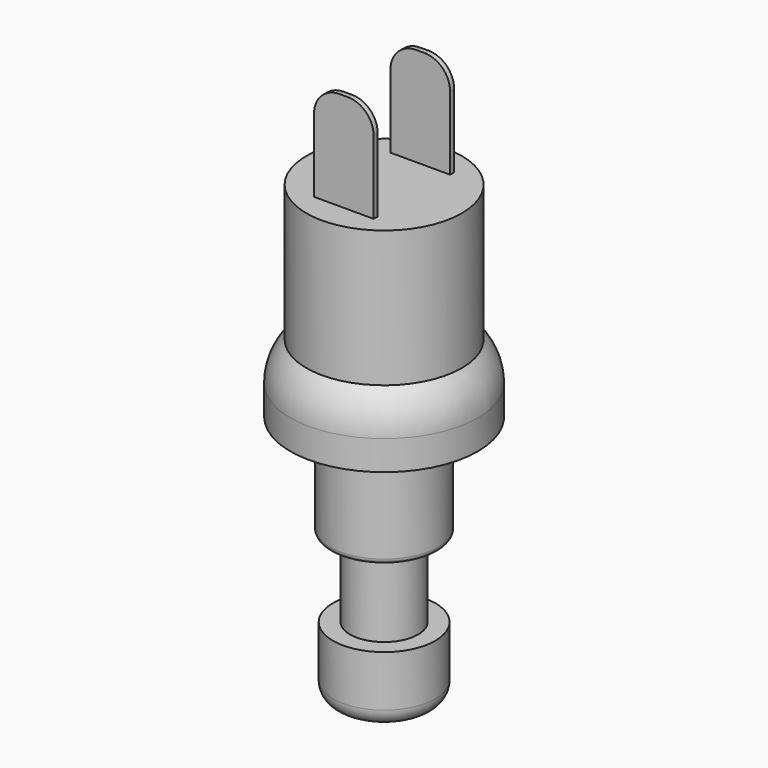
from build123d import *

# Parameters (mm, degrees)
F0_R      = 3
F1_DEPTH  = 4
F2_R      = 2
F3_DEPTH  = 4.6
F4_R      = 3.175
F5_DEPTH  = 6
F6_R      = 5.5
F7_DEPTH  = 4
F8_R      = 4.5612364212
F9_DEPTH  = 8
F11_R     = 1
F12_R     = 0.3
F13_W     = 3.5
F13_H     = 0.3
F14_DEPTH = 5.8
F15_R     = 1.5


# Not quite as in the source:
# - a fillet or chamfer that OpenCascade refuses, or shapes differently, is made with other operations: its cross-section is extruded or revolved along the edge and cut away or added


with BuildPart() as f1:
    # F0 (on Top) → F1 (new body)
    with BuildSketch(Plane.XY):
        Circle(F0_R)
    extrude(amount=F1_DEPTH)

    # F2 (on face) → F3 (join)
    with BuildSketch(Plane.XY.offset(4)):
        Circle(F2_R)
    extrude(amount=F3_DEPTH)

    # F4 (on face) → F5 (join)
    with BuildSketch(Plane.XY.offset(8.6)):
        Circle(F4_R)
    extrude(amount=F5_DEPTH)

    # F6 (on face) → F7 (join)
    with BuildSketch(Plane.XY.offset(14.6)):
        Circle(F6_R)
    extrude(amount=F7_DEPTH)

    # F8 (on face) → F9 (join)
    with BuildSketch(Plane.XY.offset(18.6)):
        Circle(F8_R)
    extrude(amount=F9_DEPTH)

    # F10: fillet of radius 3.2064860271 on 1 edges, made by hand

    # F10_s1 → F10_t2 (revolve, cut)
    with BuildSketch(Plane.XZ):
        with BuildLine():
            ThreePointArc((5.5, 16.3330664898), (5.256027516, 17.5598778645), (4.5612364212, 18.6))
            Line((4.5612364212, 18.6), (5.5, 18.6))
            Line((5.5, 18.6), (5.5, 16.3330664898))
        make_face()
    revolve(axis=Axis((0, 0, 18.6), (0, 0, 1)), mode=Mode.SUBTRACT)

    # F11
    f11_edges = [f1.edges().sort_by_distance(p)[0] for p in [
        (-3, 0, 0),
    ]]
    fillet(f11_edges, radius=F11_R)

    # F12
    f12_edges = [f1.edges().sort_by_distance(p)[0] for p in [
        (-3.175, 0, 8.6),
    ]]
    fillet(f12_edges, radius=F12_R)

    # F13 (on face) → F14 (join)
    with BuildSketch(Plane.XY.offset(26.6)):
        with Locations((0, 2.8059364047)):
            Rectangle(F13_W, F13_H)
        with Locations((0, -2.8059364047)):
            Rectangle(F13_W, F13_H)
    extrude(amount=F14_DEPTH)

    # F15
    f15_edges = [f1.edges().sort_by_distance(p)[0] for p in [
        (1.75, 2.805936, 32.4),
        (1.75, -2.805936, 32.4),
        (-1.75, -2.805936, 32.4),
        (-1.75, 2.805936, 32.4),
    ]]
    fillet(f15_edges, radius=F15_R)


solid = f1.part
